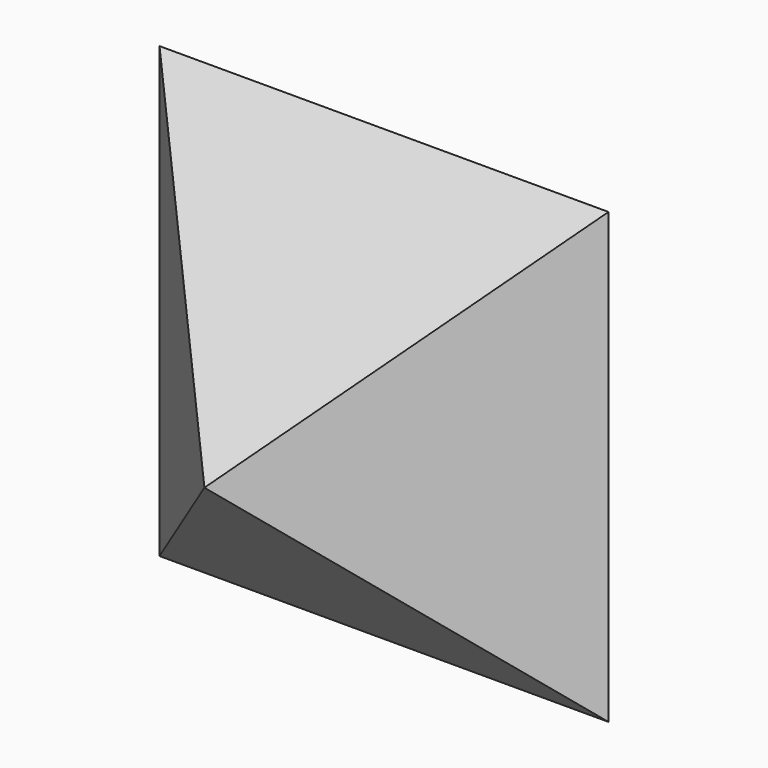
from build123d import *

# Parameters (mm, degrees)
F0_W     = 25.4
F0_H     = 25.4
F1_DEPTH = 25.4
F2_SIZE  = 12.69999
F3_W     = 25.4
F3_H     = 12.7
F4_DEPTH = 25.4


# Not quite as in the source:
# - a fillet or chamfer is up to 0.001 mm smaller than in the source, because OpenCascade refuses the exact size


with BuildPart() as f1:
    # F0 (on Front) → F1 (new body)
    with BuildSketch(Plane.XZ):
        with Locations((-12459.5173980713, 4152.3379470825)):
            Rectangle(F0_W, F0_H)
    extrude(amount=F1_DEPTH)

    # F2 (size 12.7 in the source; OpenCascade refuses exactly that, so slightly less here)
    f2_edges = [f1.edges().sort_by_distance(p)[0] for p in [
        (-12446.817398, -25.4, 4152.337947),
        (-12459.517398, -25.4, 4139.637947),
        (-12472.217398, -25.4, 4152.337947),
        (-12459.517398, -25.4, 4165.037947),
    ]]
    chamfer(f2_edges, length=F2_SIZE)

    # F3 (on face) → F4 (cut)
    with BuildSketch(Plane(origin=(0, 0, 4139.6379470825), x_dir=(1, 0, 0), z_dir=(0, 0, -1))):
        with Locations((-12459.5173980713, 6.35)):
            Rectangle(F3_W, F3_H)
    extrude(amount=-F4_DEPTH, mode=Mode.SUBTRACT)


solid = f1.part
